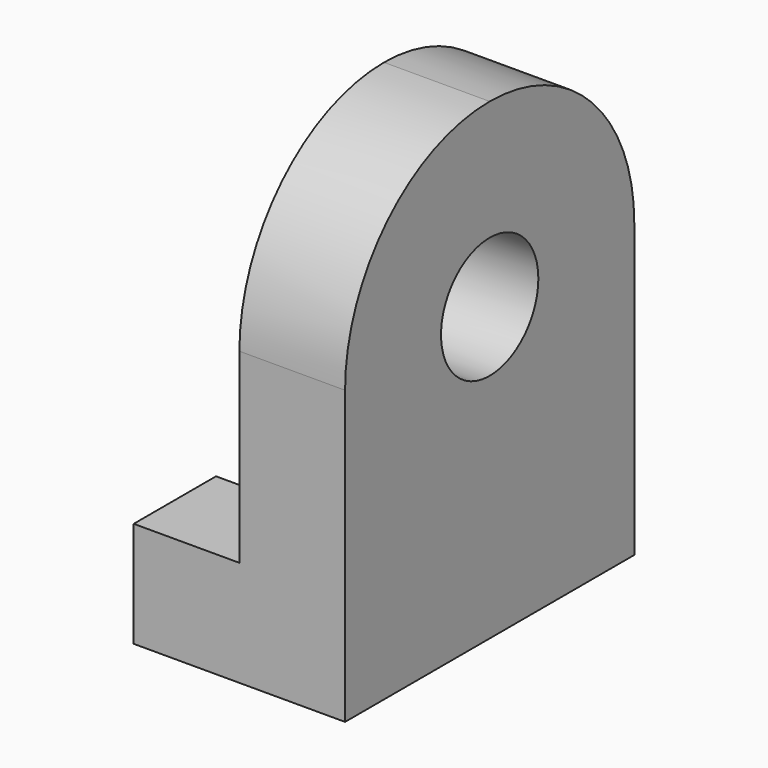
from build123d import *

# Parameters (mm, degrees)
F1_DEPTH = 66.04
F2_R     = 33.02
F3_R     = 33.01999
F4_W     = 28.448
F4_H     = 19.304
F5_DEPTH = 9.652
F6_R     = 11.1125
F7_DEPTH = 19.304


# Not quite as in the source:
# - a fillet or chamfer is up to 0.001 mm smaller than in the source, because OpenCascade refuses the exact size


with BuildPart() as f1:
    # F0 (on Front) → F1 (new body)
    with BuildSketch(Plane.XZ):
        Polygon((23.3367617899, 41.0247054291), (4.0327617899, 41.0247054291), (4.0327617899, -26.0312945709), (-15.2712382101, -26.0312945709), (-15.2712382101, -45.3352945709), (23.3367617899, -45.3352945709), align=None)
    extrude(amount=F1_DEPTH)

    # F2
    f2_edges = [f1.edges().sort_by_distance(p)[0] for p in [
        (13.684762, 0, 41.024705),
    ]]
    fillet(f2_edges, radius=F2_R)

    # F3 (radius 33.02 in the source; OpenCascade refuses exactly that, so slightly less here)
    f3_edges = [f1.edges().sort_by_distance(p)[0] for p in [
        (13.684762, -66.04, 41.024705),
    ]]
    fillet(f3_edges, radius=F3_R)

    # F4 (on face) → F5 (cut)
    with BuildSketch(Plane(origin=(-15.2712382101, 0, 0), x_dir=(0, -1, 0), z_dir=(-1, 0, 0))):
        with Locations((33.02, -35.6832945709)):
            Rectangle(F4_W, F4_H)
    extrude(amount=-F5_DEPTH, mode=Mode.SUBTRACT)

    # F6 (on face) → F7 (cut)
    with BuildSketch(Plane.YZ.offset(23.3367617899)):
        with Locations((-33.02, 8.0047054291)):
            Circle(F6_R)
    extrude(amount=-F7_DEPTH, mode=Mode.SUBTRACT)


solid = f1.part
